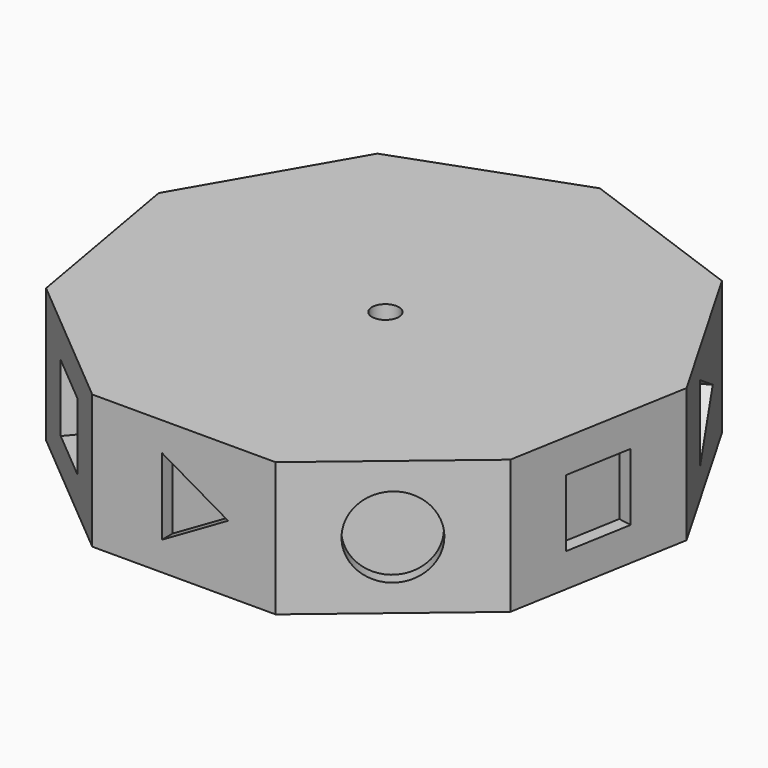
from build123d import *

# Parameters (mm, degrees)
F0_R            = 5
F1_DEPTH        = 50
F2_R            = 15
F3_DEPTH        = 5
F3_COPIES_COUNT = 3
F4_W            = 25
F4_H            = 25
F5_DEPTH        = 5
F5_COPIES_COUNT = 3
F7_DEPTH        = 5
F7_COPIES_COUNT = 3


# Not quite as in the source:
# - a pattern or mirror of a feature is missing from the dataset's text; its kind, count and spacing are read off the source's solid


with BuildPart() as f1:
    # F0 (on Top) → F1 (new body)
    with BuildSketch(Plane.XY):
        Polygon((64.2787609687, 76.6044443119), (0, 100), (-64.2787609687, 76.6044443119), (-98.4807753012, 17.3648177667), (-86.6025403784, -50), (-34.2020143326, -93.9692620786), (34.2020143326, -93.9692620786), (86.6025403784, -50), (98.4807753012, 17.3648177667), align=None)
        Circle(F0_R, mode=Mode.SUBTRACT)
    extrude(amount=F1_DEPTH)

    # F2 (on face) → F3 (cut)
    with BuildSketch(Plane(origin=(60.4022773555, -71.9846310393, 0), x_dir=(0.7660444431, 0.6427876097, 0), z_dir=(0.6427876097, -0.7660444431, 0))):
        with Locations((0, 25)):
            Circle(F2_R)
    f3 = extrude(amount=-F3_DEPTH, mode=Mode.SUBTRACT)

    # F3_copies: F3 ×3 about axis
    f3_copies_axis = Axis((0, 0, 0), (0, 0, 1))
    for i in range(1, F3_COPIES_COUNT):
        add(f3.rotate(f3_copies_axis, i * 360 / F3_COPIES_COUNT), mode=Mode.SUBTRACT)

    # F4 (on face) → F5 (cut)
    with BuildSketch(Plane(origin=(-60.4022773555, -71.9846310393, 0), x_dir=(0.7660444431, -0.6427876097, 0), z_dir=(-0.6427876097, -0.7660444431, 0))):
        with Locations((0, 25)):
            Rectangle(F4_W, F4_H)
    f5 = extrude(amount=-F5_DEPTH, mode=Mode.SUBTRACT)

    # F5_copies: F5 ×3 about axis
    f5_copies_axis = Axis((0, 0, 0), (0, 0, 1))
    for i in range(1, F5_COPIES_COUNT):
        add(f5.rotate(f5_copies_axis, i * 360 / F5_COPIES_COUNT), mode=Mode.SUBTRACT)

    # F6 (on face) → F7 (cut)
    with BuildSketch(Plane.XZ.offset(93.9692620786)):
        Polygon((-8.25, 10.7105808376), (16.5, 25), (-8.25, 39.2894191624), align=None)
    f7 = extrude(amount=-F7_DEPTH, mode=Mode.SUBTRACT)

    # F7_copies: F7 ×3 about axis
    f7_copies_axis = Axis((0, 0, 0), (0, 0, 1))
    for i in range(1, F7_COPIES_COUNT):
        add(f7.rotate(f7_copies_axis, i * 360 / F7_COPIES_COUNT), mode=Mode.SUBTRACT)


solid = f1.part
